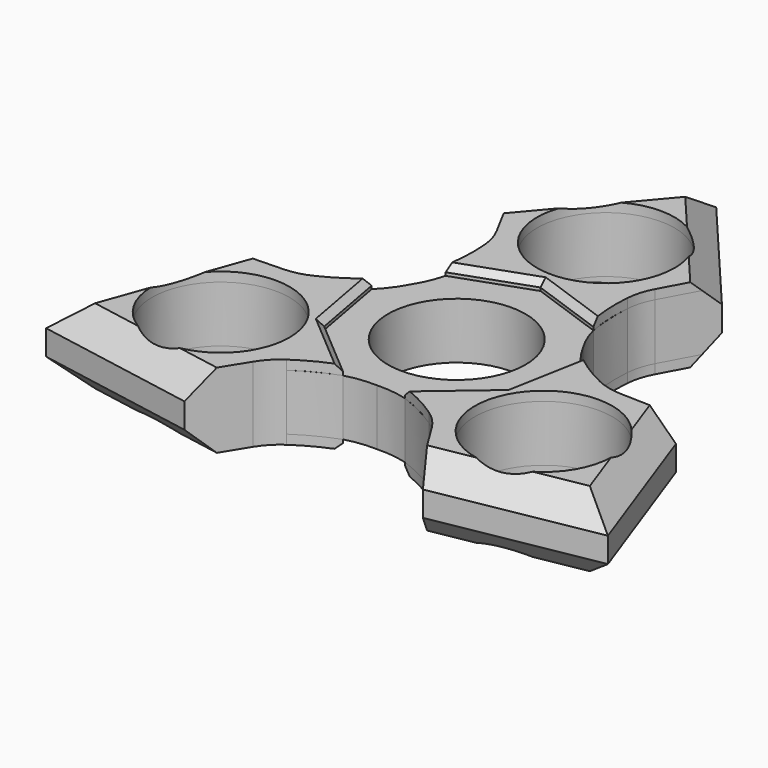
from build123d import *

# Parameters (mm, degrees)
F0_R          = 11
F1_DEPTH      = 9
F2_R          = 15.2479467251
F2_R_2        = 11
F3_DEPTH      = 9
F4_R          = 11
F5_DEPTH      = 1.5
F5_DEPTH_BACK = 10.5
F6_SIZE       = 1
F7_T1_DEPTH   = 46.8540451744
F7_T3_DEPTH   = 46.8540451744
F7_T5_DEPTH   = 46.8540451744
F7_T7_DEPTH   = 46.8540451744
F7_T9_DEPTH   = 46.8540451744
F7_T11_DEPTH  = 46.8540451744
F8_TEXT_SIZE  = 5.2253238128
F9_DEPTH      = 1


# Not quite as in the source:
# - a fillet or chamfer that OpenCascade refuses, or shapes differently, is made with other operations: its cross-section is extruded or revolved along the edge and cut away or added
# - Text() gives the source's letters only with a copy of the font that has no kerning and outlines rounded to 1/6400 em; it was checked with that copy


with BuildPart() as f1:
    # F0 (on Top) → F1 (new body)
    with BuildSketch(Plane.XY):
        with BuildLine():
            ThreePointArc((13.9107648145, 5.6116505838), (14.7251735511, 2.8581924167), (15, 0))
            ThreePointArc((15, 0), (11.323278162, -9.8378540173), (2.0955504446, -14.8529010074))
            ThreePointArc((2.0955504446, -14.8529010074), (1.796918769, -14.8919804908), (1.497562671, -14.9250563164))
            ThreePointArc((1.497562671, -14.9250563164), (0.7472925834, -15.0329595481), (0, -15.1598536248))
            ThreePointArc((0, -15.1598536248), (2.5052648491, -15.7302865484), (4.9522810052, -16.5137772097))
            ThreePointArc((4.9522810052, -16.5137772097), (8.2735998473, -17.9714764747), (11.3938909721, -19.8207545212))
            ThreePointArc((11.3938909721, -19.8207545212), (13.0052870701, -21.1818254362), (14.2953482889, -22.8506134609))
            Line((14.2953482889, -22.8506134609), (19.0779680509, -30.6088705205))
            Line((19.0779680509, -30.6088705205), (44.9417915182, -25.9471554309))
            Line((44.9417915182, -25.9471554309), (36.0470434774, -1.2175697244))
            Line((36.0470434774, -1.2175697244), (26.9368858937, -0.9548280437))
            ThreePointArc((26.9368858937, -0.9548280437), (24.8466424613, -0.6719962681), (22.8622224236, 0.0429782308))
            ThreePointArc((22.8622224236, 0.0429782308), (19.7005550942, 1.8205905889), (16.7774910786, 3.9680874476))
            ThreePointArc((16.7774910786, 3.9680874476), (14.8754601843, 5.6955202716), (13.1288183568, 7.5799268124))
            ThreePointArc((13.1288183568, 7.5799268124), (13.3925711544, 6.8693054128), (13.6742592584, 6.1656008413))
            ThreePointArc((13.6742592584, 6.1656008413), (13.7952928022, 5.8898129429), (13.9107648145, 5.6116505838))
        make_face()
        with Locations((25.82601704, -14.9106578901)):
            Circle(F0_R, mode=Mode.SUBTRACT)
        with BuildLine():
            ThreePointArc((11.81521437, 9.2412504236), (11.9983740332, 9.0021675479), (12.1766965874, 8.759455475))
            ThreePointArc((12.1766965874, 8.759455475), (12.645278571, 8.1636541353), (13.1288183568, 7.5799268124))
            ThreePointArc((13.1288183568, 7.5799268124), (12.3701953351, 10.0347662768), (11.8252100734, 12.5456897621))
            ThreePointArc((11.8252100734, 12.5456897621), (11.426955247, 16.1508858858), (11.4683314515, 19.7777762904))
            ThreePointArc((11.4683314515, 19.7777762904), (11.8413553912, 21.8538217043), (12.6415376048, 23.8054415046))
            Line((12.6415376048, 23.8054415046), (16.9690754265, 31.8264402449))
            Line((16.9690754265, 31.8264402449), (0, 51.8943108618))
            Line((0, 51.8943108618), (-16.9690754265, 31.8264402449))
            Line((-16.9690754265, 31.8264402449), (-12.6415376048, 23.8054415046))
            ThreePointArc((-12.6415376048, 23.8054415046), (-11.8413553912, 21.8538217043), (-11.4683314515, 19.7777762904))
            ThreePointArc((-11.4683314515, 19.7777762904), (-11.426955247, 16.1508858858), (-11.8252100734, 12.5456897621))
            ThreePointArc((-11.8252100734, 12.5456897621), (-12.3701953351, 10.0347662768), (-13.1288183568, 7.5799268124))
            ThreePointArc((-13.1288183568, 7.5799268124), (-12.645278571, 8.1636541353), (-12.1766965874, 8.759455475))
            ThreePointArc((-12.1766965874, 8.759455475), (-11.9983740332, 9.0021675479), (-11.81521437, 9.2412504236))
            ThreePointArc((-11.81521437, 9.2412504236), (0, 15), (11.81521437, 9.2412504236))
        make_face()
        with Locations((0, 29.8213157803)):
            Circle(F0_R, mode=Mode.SUBTRACT)
        with BuildLine():
            ThreePointArc((11.8252100734, 12.5456897621), (12.3701953351, 10.0347662768), (13.1288183568, 7.5799268124))
            ThreePointArc((13.1288183568, 7.5799268124), (14.8754601843, 5.6955202716), (16.7774910786, 3.9680874476))
            ThreePointArc((16.7774910786, 3.9680874476), (15.1368369171, 5.8545979838), (13.8023376862, 7.9687833786))
            ThreePointArc((13.8023376862, 7.9687833786), (12.6386490415, 10.1815863113), (11.8252100734, 12.5456897621))
        make_face()
        with BuildLine():
            ThreePointArc((0, -15.1598536248), (-0.7472925834, -15.0329595481), (-1.497562671, -14.9250563164))
            ThreePointArc((-1.497562671, -14.9250563164), (-1.796918769, -14.8919804908), (-2.0955504446, -14.8529010074))
            ThreePointArc((-2.0955504446, -14.8529010074), (-12.9903810568, -7.5), (-13.9107648145, 5.6116505838))
            ThreePointArc((-13.9107648145, 5.6116505838), (-13.7952928022, 5.8898129429), (-13.6742592584, 6.1656008413))
            ThreePointArc((-13.6742592584, 6.1656008413), (-13.3925711544, 6.8693054128), (-13.1288183568, 7.5799268124))
            ThreePointArc((-13.1288183568, 7.5799268124), (-14.8754601843, 5.6955202716), (-16.7774910786, 3.9680874476))
            ThreePointArc((-16.7774910786, 3.9680874476), (-19.7005550942, 1.8205905889), (-22.8622224236, 0.0429782308))
            ThreePointArc((-22.8622224236, 0.0429782308), (-24.8466424613, -0.6719962681), (-26.9368858937, -0.9548280437))
            Line((-26.9368858937, -0.9548280437), (-36.0470434774, -1.2175697244))
            Line((-36.0470434774, -1.2175697244), (-44.9417915182, -25.9471554309))
            Line((-44.9417915182, -25.9471554309), (-19.0779680509, -30.6088705205))
            Line((-19.0779680509, -30.6088705205), (-14.2953482889, -22.8506134609))
            ThreePointArc((-14.2953482889, -22.8506134609), (-13.0052870701, -21.1818254362), (-11.3938909721, -19.8207545212))
            ThreePointArc((-11.3938909721, -19.8207545212), (-8.2735998473, -17.9714764747), (-4.9522810052, -16.5137772097))
            ThreePointArc((-4.9522810052, -16.5137772097), (-2.5052648491, -15.7302865484), (0, -15.1598536248))
        make_face()
        with Locations((-25.82601704, -14.9106578901)):
            Circle(F0_R, mode=Mode.SUBTRACT)
        with BuildLine():
            ThreePointArc((4.9522810052, -16.5137772097), (2.5052648491, -15.7302865484), (0, -15.1598536248))
            ThreePointArc((0, -15.1598536248), (-2.5052648491, -15.7302865484), (-4.9522810052, -16.5137772097))
            ThreePointArc((-4.9522810052, -16.5137772097), (-2.4981878756, -16.0361842951), (0, -15.9375667572))
            ThreePointArc((0, -15.9375667572), (2.4981878756, -16.0361842951), (4.9522810052, -16.5137772097))
        make_face()
        with BuildLine():
            ThreePointArc((-16.7774910786, 3.9680874476), (-14.8754601843, 5.6955202716), (-13.1288183568, 7.5799268124))
            ThreePointArc((-13.1288183568, 7.5799268124), (-12.3701953351, 10.0347662768), (-11.8252100734, 12.5456897621))
            ThreePointArc((-11.8252100734, 12.5456897621), (-12.6386490415, 10.1815863113), (-13.8023376862, 7.9687833786))
            ThreePointArc((-13.8023376862, 7.9687833786), (-15.1368369171, 5.8545979838), (-16.7774910786, 3.9680874476))
        make_face()
    extrude(amount=F1_DEPTH)

    # F2 (on face) → F3 (join)
    with BuildSketch(Plane.XY.offset(9)):
        Circle(F2_R)
        Circle(F2_R_2, mode=Mode.SUBTRACT)
    extrude(amount=-F3_DEPTH)

    # F4 (on face) → F5 (join, two sides)
    with BuildSketch(Plane.XY.offset(9)) as f5_sk:
        with BuildLine():
            Line((-26.9368858937, -0.9548280437), (-36.0470434774, -1.2175697244))
            Line((-36.0470434774, -1.2175697244), (-44.9417915182, -25.9471554309))
            Line((-44.9417915182, -25.9471554309), (-19.0779680509, -30.6088705205))
            Line((-19.0779680509, -30.6088705205), (-14.2953482889, -22.8506134609))
            ThreePointArc((-14.2953482889, -22.8506134609), (-13.0052870701, -21.1818254362), (-11.3938909721, -19.8207545212))
            ThreePointArc((-11.3938909721, -19.8207545212), (-8.2804771911, -17.9580802029), (-4.9522810052, -16.5137772097))
            Line((-4.9522810052, -16.5137772097), (-14.5024295496, -8.3729816043))
            Line((-14.5024295496, -8.3729816043), (-16.7774910786, 3.9680874476))
            ThreePointArc((-16.7774910786, 3.9680874476), (-19.6923922545, 1.8079364985), (-22.8622224236, 0.0429782308))
            ThreePointArc((-22.8622224236, 0.0429782308), (-24.8466424613, -0.6719962681), (-26.9368858937, -0.9548280437))
        make_face()
        with Locations((-25.82601704, -14.9106578901)):
            Circle(F4_R, mode=Mode.SUBTRACT)
        with BuildLine():
            Line((14.2953482889, -22.8506134609), (19.0779680509, -30.6088705205))
            Line((19.0779680509, -30.6088705205), (44.9417915182, -25.9471554309))
            Line((44.9417915182, -25.9471554309), (36.0470434774, -1.2175697244))
            Line((36.0470434774, -1.2175697244), (26.9368858937, -0.9548280437))
            ThreePointArc((26.9368858937, -0.9548280437), (24.8466424613, -0.6719962681), (22.8622224236, 0.0429782308))
            ThreePointArc((22.8622224236, 0.0429782308), (19.6923922545, 1.8079364985), (16.7774910786, 3.9680874476))
            Line((16.7774910786, 3.9680874476), (14.5024295496, -8.3729816043))
            Line((14.5024295496, -8.3729816043), (4.9522810052, -16.5137772097))
            ThreePointArc((4.9522810052, -16.5137772097), (8.2804771911, -17.9580802029), (11.3938909721, -19.8207545212))
            ThreePointArc((11.3938909721, -19.8207545212), (13.0052870701, -21.1818254362), (14.2953482889, -22.8506134609))
        make_face()
        with Locations((25.82601704, -14.9106578901)):
            Circle(F4_R, mode=Mode.SUBTRACT)
        with BuildLine():
            Line((12.6415376048, 23.8054415046), (16.9690754265, 31.8264402449))
            Line((16.9690754265, 31.8264402449), (0, 51.8943108618))
            Line((0, 51.8943108618), (-16.9690754265, 31.8264402449))
            Line((-16.9690754265, 31.8264402449), (-12.6415376048, 23.8054415046))
            ThreePointArc((-12.6415376048, 23.8054415046), (-11.8413553912, 21.8538217043), (-11.4683314515, 19.7777762904))
            ThreePointArc((-11.4683314515, 19.7777762904), (-11.4119150633, 16.1501437044), (-11.8252100734, 12.5456897621))
            Line((-11.8252100734, 12.5456897621), (0, 16.7459632087))
            Line((0, 16.7459632087), (11.8252100734, 12.5456897621))
            ThreePointArc((11.8252100734, 12.5456897621), (11.4119150633, 16.1501437044), (11.4683314515, 19.7777762904))
            ThreePointArc((11.4683314515, 19.7777762904), (11.8413553912, 21.8538217043), (12.6415376048, 23.8054415046))
        make_face()
        with Locations((0, 29.8213157803)):
            Circle(F4_R, mode=Mode.SUBTRACT)
    extrude(amount=F5_DEPTH)
    extrude(f5_sk.sketch, amount=-F5_DEPTH_BACK)

    # F6
    f6_edges = [f1.edges().sort_by_distance(p)[0] for p in [
        (-15.63996, -2.202447, 10.5),
        (-9.727355, -12.443379, 10.5),
        (-9.727355, -12.443379, -1.5),
        (-15.63996, -2.202447, -1.5),
        (9.727355, -12.443379, -1.5),
        (15.63996, -2.202447, -1.5),
        (5.912605, 14.645826, -1.5),
        (-5.912605, 14.645826, -1.5),
        (15.63996, -2.202447, 10.5),
        (9.727355, -12.443379, 10.5),
        (5.912605, 14.645826, 10.5),
        (-5.912605, 14.645826, 10.5),
    ]]
    chamfer(f6_edges, length=F6_SIZE)

    # F7: chamfer of 4 on 12 edges, made by hand

    # F7_s2 → F7_t1 (cut)
    with BuildSketch(Plane(origin=(-49.1217395582, 8.8537394641, 0), x_dir=(0, 0, 1), z_dir=(0.9841419869, -0.1773824955, 0))):
        Polygon((10.5, 29.5075722317), (6.5, 33.5075722317), (10.5, 33.5075722317), align=None)
        Polygon((-1.5, 29.5075722317), (2.5, 33.5075722317), (-1.5, 33.5075722317), align=None)
    extrude(amount=F7_T1_DEPTH, mode=Mode.SUBTRACT)

    # F7_s4 → F7_t3 (cut)
    with BuildSketch(Plane(origin=(-1.0354028017, -2.8786742703, 0), x_dir=(0, 0, 1), z_dir=(-0.3384532461, -0.9409832093, 0))):
        Polygon((10.5, 29.5075722317), (6.5, 33.5075722317), (10.5, 33.5075722317), align=None)
        Polygon((-1.5, 29.5075722317), (2.5, 33.5075722317), (-1.5, 33.5075722317), align=None)
    extrude(amount=F7_T3_DEPTH, mode=Mode.SUBTRACT)

    # F7_s6 → F7_t5 (cut)
    with BuildSketch(Plane(origin=(3.0107064482, 0.5426520057, 0), x_dir=(0, 0, 1), z_dir=(0.9841419869, 0.1773824955, 0))):
        Polygon((10.5, 29.5075722317), (6.5, 33.5075722317), (10.5, 33.5075722317), align=None)
        Polygon((-1.5, 29.5075722317), (2.5, 33.5075722317), (-1.5, 33.5075722317), align=None)
    extrude(amount=F7_T5_DEPTH, mode=Mode.SUBTRACT)

    # F7_s8 → F7_t7 (cut)
    with BuildSketch(Plane(origin=(16.8933064847, -46.9675440675, 0), x_dir=(0, 0, 1), z_dir=(-0.3384532461, 0.9409832093, 0))):
        Polygon((10.5, 29.5075722317), (6.5, 33.5075722317), (10.5, 33.5075722317), align=None)
        Polygon((-1.5, 29.5075722317), (2.5, 33.5075722317), (-1.5, 33.5075722317), align=None)
    extrude(amount=F7_T7_DEPTH, mode=Mode.SUBTRACT)

    # F7_s10 → F7_t9 (cut)
    with BuildSketch(Plane(origin=(-1.9753036465, 2.3360222646, 0), x_dir=(0, 0, 1), z_dir=(-0.6456887407, 0.7636007138, 0))):
        Polygon((10.5, 29.5075722317), (6.5, 33.5075722317), (10.5, 33.5075722317), align=None)
        Polygon((2.5, 33.5075722317), (-1.5, 29.5075722317), (-1.5, 33.5075722317), align=None)
    extrude(amount=F7_T9_DEPTH, mode=Mode.SUBTRACT)

    # F7_s12 → F7_t11 (cut)
    with BuildSketch(Plane(origin=(32.2284330735, 38.1138046034, 0), x_dir=(0, 0, 1), z_dir=(-0.6456887407, -0.7636007138, 0))):
        Polygon((2.5, 33.5075722317), (-1.5, 29.5075722317), (-1.5, 33.5075722317), align=None)
        Polygon((10.5, 29.5075722317), (6.5, 33.5075722317), (10.5, 33.5075722317), align=None)
    extrude(amount=F7_T11_DEPTH, mode=Mode.SUBTRACT)

    # F8 (on face) → F9 (cut)
    with BuildSketch(Plane(origin=(0, 0, 0), x_dir=(1, 0, 0), z_dir=(0, 0, -1))):
        with Locations((-3.5476655603, -15.4858447535)):
            Text('CD', F8_TEXT_SIZE, font='Open Sans', text_align=(TextAlign.LEFT, TextAlign.BOTTOM))
    extrude(amount=-F9_DEPTH, mode=Mode.SUBTRACT)


solid = f1.part
